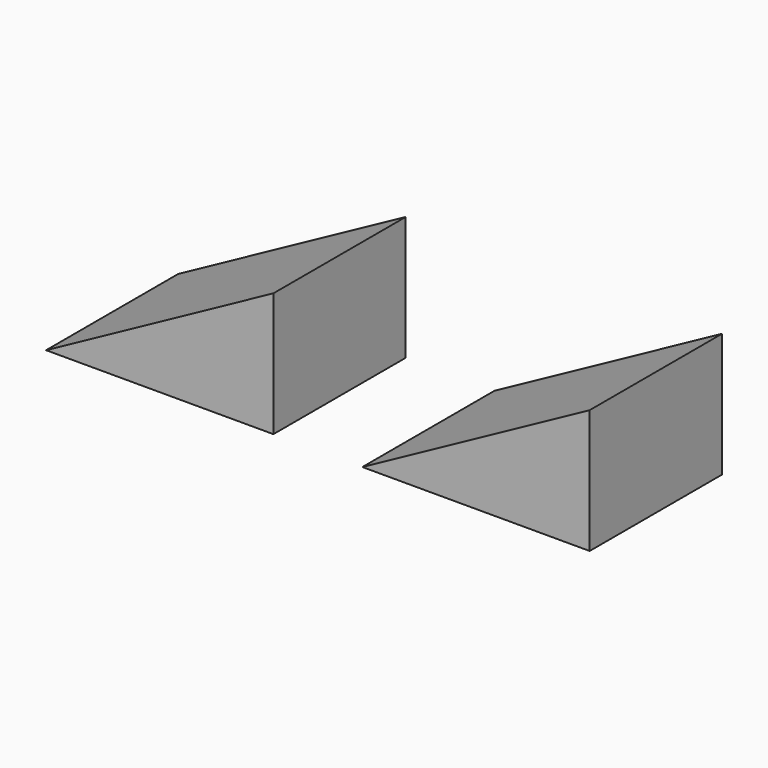
from build123d import *

# Parameters (mm, degrees)
F1_DEPTH = 40


# Not quite as in the source:
# - a feature names something its author has since deleted; it is built from what else it names


with BuildPart() as f1:
    # F0 (on Front) → F1 (new body)
    with BuildSketch(Plane.XZ):
        Polygon((56.6261941055, -11.017032899), (56.6261941055, 18.982967101), (1.6261941055, -11.017032899), align=None)
    extrude(amount=F1_DEPTH)


with BuildPart() as f1b:
    # F0 (on Front) → F1, piece 2 (new body)
    with BuildSketch(Plane.XZ):
        Polygon((133.1447663903, 18.982967101), (78.1447663903, -11.017032899), (133.1447663903, -11.017032899), align=None)
    extrude(amount=F1_DEPTH)


solid = Compound([f1.part, f1b.part])
